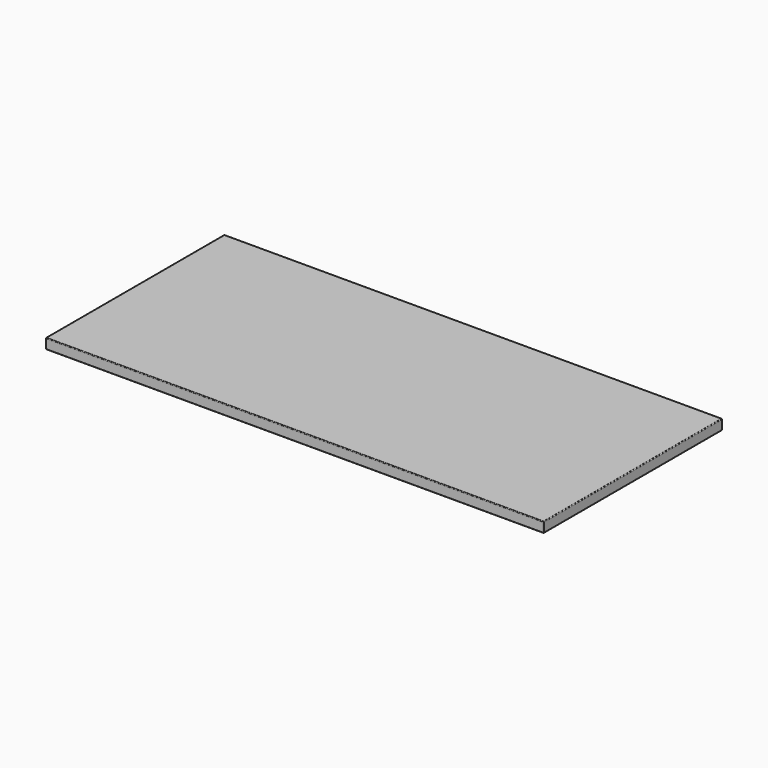
from build123d import *

# Parameters (mm, degrees)
F0_W     = 1450
F0_H     = 650
F1_DEPTH = 30
F2_R     = 2
F3_W     = 1386
F3_H     = 586
F4_DEPTH = 25
F5_R     = 5


with BuildPart() as f1:
    # F0 (on Top) → F1 (new body)
    with BuildSketch(Plane.XY):
        with Locations((725, 325)):
            Rectangle(F0_W, F0_H)
    extrude(amount=-F1_DEPTH)

    # F2
    f2_edges = [f1.edges().sort_by_distance(p)[0] for p in [
        (0, 650, -15),
        (725, 650, -30),
        (0, 325, -30),
        (725, 0, -30),
        (1450, 325, -30),
        (0, 325, 0),
        (725, 0, 0),
        (1450, 325, 0),
        (725, 650, 0),
        (0, 0, -15),
        (1450, 0, -15),
        (1450, 650, -15),
    ]]
    fillet(f2_edges, radius=F2_R)

    # F3 (on face) → F4 (cut)
    with BuildSketch(Plane(origin=(0, 0, -30), x_dir=(1, 0, 0), z_dir=(0, 0, -1))):
        with Locations((725, -325)):
            Rectangle(F3_W, F3_H)
    extrude(amount=-F4_DEPTH, mode=Mode.SUBTRACT)

    # F5
    f5_edges = [f1.edges().sort_by_distance(p)[0] for p in [
        (1418, 618, -17.5),
        (1418, 32, -17.5),
        (32, 32, -17.5),
        (32, 325, -30),
        (1418, 325, -30),
        (32, 618, -17.5),
        (725, 618, -30),
        (725, 32, -30),
    ]]
    fillet(f5_edges, radius=F5_R)


solid = f1.part
